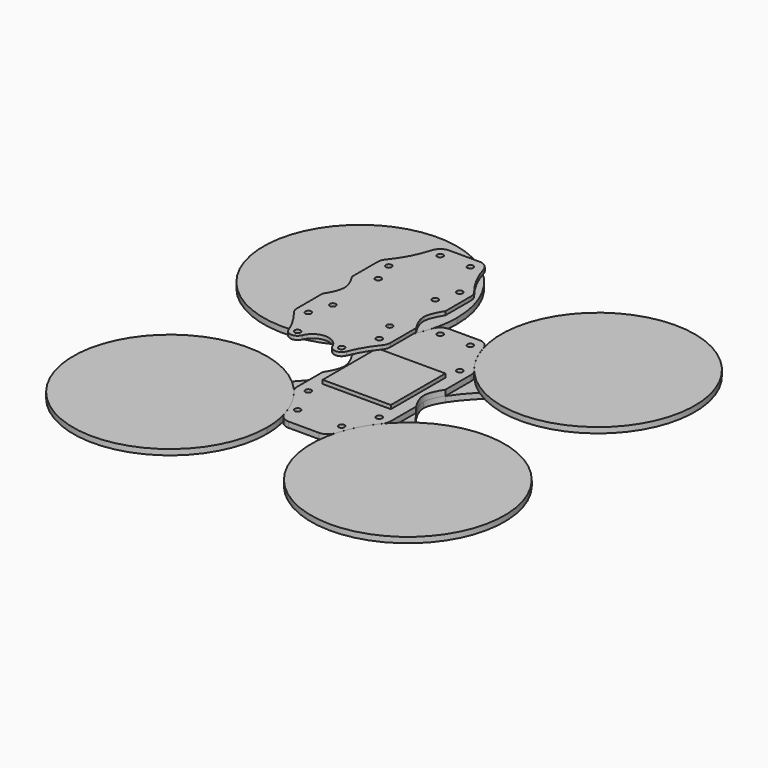
from build123d import *
from build123d import SkipClean  # not in build123d's __all__

# Parameters (mm, degrees)
F0_W      = 36.5
F0_H      = 20.4291760919
F0_H_2    = 36.5
F1_DEPTH  = 3
F2_DEPTH  = 5
F3_DEPTH  = 3
F5_DEPTH  = 3
F6_R      = 6
F8_DEPTH  = 3.001
F9_COUNT  = 2
F9_ANGLE  = 180
F12_DEPTH = 6.0010001
F14_R     = 1.6
F15_DEPTH = 6.0010001
F16_R     = 1.6
F17_DEPTH = 2
F20_DEPTH = 43.0010001


# Not quite as in the source:
# - the dataset's text gives a spline's control points without its knots; the knots are read off the source's solid
# - a pattern or mirror of a feature is missing from the dataset's text; its kind, count and spacing are read off the source's solid


with BuildPart() as f1:
    # F0 (on Top) → F1 (new body)
    with BuildSketch(Plane.XY):
        with BuildLine():
            ThreePointArc((18.25, 38.6791760919), (14.9470579592, 45.9682960976), (12.8062575721, 53.6791760919))
            Line((12.8062575721, 53.6791760919), (-12.8062575721, 53.6791760919))
            ThreePointArc((-12.8062575721, 53.6791760919), (-14.9470579592, 45.9682960976), (-18.25, 38.6791760919))
            Line((-18.25, 38.6791760919), (18.25, 38.6791760919))
        make_face()
        with Locations((0, 28.4645880459)):
            Rectangle(F0_W, F0_H)
        Rectangle(F0_W, F0_H_2)
        with Locations((0, -28.4645880459)):
            Rectangle(F0_W, F0_H)
        with BuildLine():
            ThreePointArc((12.8062575721, -53.6791760919), (14.9470579592, -45.9682960976), (18.25, -38.6791760919))
            Line((18.25, -38.6791760919), (-18.25, -38.6791760919))
            ThreePointArc((-18.25, -38.6791760919), (-14.9470579592, -45.9682960976), (-12.8062575721, -53.6791760919))
            Line((-12.8062575721, -53.6791760919), (12.8062575721, -53.6791760919))
        make_face()
        with BuildLine():
            Line((-18.25, 18.25), (-18.25, 38.6791760919))
            ThreePointArc((-18.25, 38.6791760919), (-21.3551418827, 33.7186522658), (-25, 29.1400376234))
            Line((-25, 29.1400376234), (-25, -29.1400376234))
            ThreePointArc((-25, -29.1400376234), (-21.3551418827, -33.7186522658), (-18.25, -38.6791760919))
            Line((-18.25, -38.6791760919), (-18.25, -18.25))
            Line((-18.25, -18.25), (-18.25, 18.25))
        make_face()
        with BuildLine():
            Line((25, -29.1400376234), (25, 29.1400376234))
            ThreePointArc((25, 29.1400376234), (21.3551418827, 33.7186522658), (18.25, 38.6791760919))
            Line((18.25, 38.6791760919), (18.25, 18.25))
            Line((18.25, 18.25), (18.25, -18.25))
            Line((18.25, -18.25), (18.25, -38.6791760919))
            ThreePointArc((18.25, -38.6791760919), (21.3551418827, -33.7186522658), (25, -29.1400376234))
        make_face()
    extrude(amount=F1_DEPTH)

    # F6
    f6_edges = [f1.edges().sort_by_distance(p)[0] for p in [
        (25, -29.140038, 1.5),
        (12.806258, -53.679176, 1.5),
        (25, 29.140038, 1.5),
        (12.806258, 53.679176, 1.5),
        (-12.806258, 53.679176, 1.5),
        (-25, 29.140038, 1.5),
        (-25, -29.140038, 1.5),
        (-12.806258, -53.679176, 1.5),
    ]]
    fillet(f6_edges, radius=F6_R)

    # F11 (on face) → F12 (cut, through all)
    with BuildSketch(Plane.XY.offset(3)):
        with BuildLine():
            Line((-25, 9.7909347539), (-25, -9.7909347533))
            add(Edge.make_bspline(
                [(-21.2132034356, 0), (-21.2132034356, -2.8448051924), (-22.673791932, -6.2126162774), (-24.9999999996, -9.7909347533)],
                knots=[0, 0, 0, 0, 0.1869288415, 0.1869288415, 0.1869288415, 0.1869288415], degree=3))
            add(Edge.make_bspline(
                [(-21.2132034356, 0), (-21.2132034356, 2.8448051925), (-22.6737919322, 6.2126162777), (-25, 9.7909347539)],
                knots=[0, 0, 0, 0, 0.1869288415, 0.1869288415, 0.1869288415, 0.1869288415], degree=3))
        make_face()
        with BuildLine():
            add(Edge.make_bspline(
                [(21.2132034356, 0), (21.2132034356, 2.8448051924), (22.673791932, 6.2126162774), (24.9999999996, 9.7909347533)],
                knots=[0, 0, 0, 0, 0.1869288415, 0.1869288415, 0.1869288415, 0.1869288415], degree=3))
            add(Edge.make_bspline(
                [(21.2132034356, 0), (21.2132034356, -2.8448051925), (22.6737919322, -6.2126162777), (25, -9.7909347539)],
                knots=[0, 0, 0, 0, 0.1869288415, 0.1869288415, 0.1869288415, 0.1869288415], degree=3))
            Line((25, -9.7909347539), (25, 9.7909347533))
        make_face()
    extrude(amount=-F12_DEPTH, mode=Mode.SUBTRACT)

    # F14 (on face) → F15 (cut, through all)
    with BuildSketch(Plane.XY.offset(3)):
        with Locations((19, 26.9225135853)):
            Circle(F14_R)
        with Locations((19, -26.9225135853)):
            Circle(F14_R)
        with Locations((8.0868917444, 47.6791760919)):
            Circle(F14_R)
        with Locations((15.25, 15.25)):
            Circle(F14_R)
        with Locations((15.25, -15.25)):
            Circle(F14_R)
        with Locations((11.7638554054, -43.0836852872)):
            Circle(F14_R)
    f15 = extrude(amount=-F15_DEPTH, mode=Mode.SUBTRACT)

    # F15_copies: F15 across plane
    add(f15.mirror(Plane(origin=(0, 0, 0), x_dir=(0, 0, -1), z_dir=(-1, 0, 0))), clean=False, mode=Mode.SUBTRACT)


with BuildPart() as f2:
    # F0 (on Top) → F2 (new body)
    with BuildSketch(Plane.XY):
        Rectangle(F0_W, F0_H_2)
    extrude(amount=F2_DEPTH)


with BuildPart() as f3:
    # F0 (on Top) → F3 (new body)
    with BuildSketch(Plane.XY):
        with BuildLine():
            Line((-25, 53.6791760919), (-12.8062575721, 53.6791760919))
            ThreePointArc((-12.8062575721, 53.6791760919), (-12.0818384792, 58.6359951966), (-11.8396103068, 63.6396103068))
            ThreePointArc((-11.8396103068, 63.6396103068), (-112.0378117914, 82.1018445447), (-25, 29.1400376234))
            Line((-25, 29.1400376234), (-25, 53.6791760919))
        make_face()
        with BuildLine():
            ThreePointArc((-18.25, 38.6791760919), (-14.9470579592, 45.9682960976), (-12.8062575721, 53.6791760919))
            Line((-12.8062575721, 53.6791760919), (-25, 53.6791760919))
            Line((-25, 53.6791760919), (-25, 29.1400376234))
            ThreePointArc((-25, 29.1400376234), (-21.3551418827, 33.7186522658), (-18.25, 38.6791760919))
        make_face()
    extrude(amount=F3_DEPTH)


with BuildPart() as f3b:
    # F0 (on Top) → F3, piece 2 (new body)
    with BuildSketch(Plane.XY):
        with BuildLine():
            ThreePointArc((25, 29.1400376234), (82.1018445447, 15.2414088222), (115.4396103068, 63.6396103068))
            ThreePointArc((115.4396103068, 63.6396103068), (58.6359951966, 115.1973821344), (12.8062575721, 53.6791760919))
            Line((12.8062575721, 53.6791760919), (25, 53.6791760919))
            Line((25, 53.6791760919), (25, 29.1400376234))
        make_face()
        with BuildLine():
            Line((25, 53.6791760919), (12.8062575721, 53.6791760919))
            ThreePointArc((12.8062575721, 53.6791760919), (14.9470579592, 45.9682960976), (18.25, 38.6791760919))
            ThreePointArc((18.25, 38.6791760919), (21.3551418827, 33.7186522658), (25, 29.1400376234))
            Line((25, 29.1400376234), (25, 53.6791760919))
        make_face()
    extrude(amount=F3_DEPTH)


with BuildPart() as f3c:
    # F0 (on Top) → F3, piece 3 (new body)
    with BuildSketch(Plane.XY):
        with BuildLine():
            Line((-25, -53.6791760919), (-25, -29.1400376234))
            ThreePointArc((-25, -29.1400376234), (-112.0378117914, -82.1018445447), (-11.8396103068, -63.6396103068))
            ThreePointArc((-11.8396103068, -63.6396103068), (-12.0818384792, -58.6359951966), (-12.8062575721, -53.6791760919))
            Line((-12.8062575721, -53.6791760919), (-25, -53.6791760919))
        make_face()
        with BuildLine():
            ThreePointArc((-12.8062575721, -53.6791760919), (-14.9470579592, -45.9682960976), (-18.25, -38.6791760919))
            ThreePointArc((-18.25, -38.6791760919), (-21.3551418827, -33.7186522658), (-25, -29.1400376234))
            Line((-25, -29.1400376234), (-25, -53.6791760919))
            Line((-25, -53.6791760919), (-12.8062575721, -53.6791760919))
        make_face()
    extrude(amount=F3_DEPTH)


with BuildPart() as f3d:
    # F0 (on Top) → F3, piece 4 (new body)
    with BuildSketch(Plane.XY):
        with BuildLine():
            ThreePointArc((115.4396103068, -63.6396103068), (82.1018445447, -15.2414088222), (25, -29.1400376234))
            Line((25, -29.1400376234), (25, -53.6791760919))
            Line((25, -53.6791760919), (12.8062575721, -53.6791760919))
            ThreePointArc((12.8062575721, -53.6791760919), (58.6359951966, -115.1973821344), (115.4396103068, -63.6396103068))
        make_face()
        with BuildLine():
            Line((25, -53.6791760919), (25, -29.1400376234))
            ThreePointArc((25, -29.1400376234), (21.3551418827, -33.7186522658), (18.25, -38.6791760919))
            ThreePointArc((18.25, -38.6791760919), (14.9470579592, -45.9682960976), (12.8062575721, -53.6791760919))
            Line((12.8062575721, -53.6791760919), (25, -53.6791760919))
        make_face()
    extrude(amount=F3_DEPTH)


with BuildPart() as f5:
    # F4 (on face) → F5 (new body)
    with BuildSketch(Plane.XY):
        with BuildLine():
            ThreePointArc((53.033008589, -74.2462120246), (74.2462120246, -74.2462120246), (74.2462120246, -53.033008589))
            Line((74.2462120246, -53.033008589), (21.2132034356, 0))
            Line((21.2132034356, 0), (0, 0))
            Line((0, 0), (0, -21.2132034356))
            Line((0, -21.2132034356), (53.033008589, -74.2462120246))
        make_face()
    extrude(amount=-F5_DEPTH)

    # F7 (on face) → F8 (cut, through all)
    with BuildSketch(Plane.XY):
        with BuildLine():
            add(Edge.make_bspline(
                [(25, -9.7909347539), (28.6766596733, -15.4466021988), (44.7457233208, -32.458147319), (59.4005470216, -44.1078131673), (70.4054520123, -50.2521764221)],
                knots=[0.1869288415, 0.1869288415, 0.1869288415, 0.1869288415, 0.4823769326, 1, 1, 1, 1], degree=3))
            ThreePointArc((70.4054520123, -50.2521764221), (72.4364111178, -51.4898656391), (74.2462120246, -53.033008589))
            Line((74.2462120246, -53.033008589), (25, -3.7867965644))
            Line((25, -3.7867965644), (25, -9.7909347539))
        make_face()
        with BuildLine():
            add(Edge.make_bspline(
                [(21.2132034356, 0), (21.2132034356, -2.8448051925), (22.6737919322, -6.2126162777), (25, -9.7909347539)],
                knots=[0, 0, 0, 0, 0.1869288415, 0.1869288415, 0.1869288415, 0.1869288415], degree=3))
            Line((25, -9.7909347539), (25, -3.7867965644))
            Line((25, -3.7867965644), (21.2132034356, 0))
        make_face()
    with SkipClean():  # cleaning this boolean's faces spoils the solid; the shape is the same uncleaned
        extrude(amount=-F8_DEPTH, mode=Mode.SUBTRACT)


with BuildPart() as f9_1:
    # F9: instance of F5
    add(f5.part.rotate(Axis((0, 0, -1.5), (0, 0, 1)), 1 * F9_ANGLE / (F9_COUNT - 1)), clean=False)


with BuildPart() as f10_1:
    # F10: instance of F9_1
    add(f9_1.part.mirror(Plane.YZ), clean=False)


with BuildPart() as f10_2:
    # F10: instance of F5
    add(f5.part.mirror(Plane.YZ), clean=False)


with BuildPart() as f17:
    # F16 (on offset) → F17 (new body)
    with BuildSketch(Plane.XY.offset(38)):
        with BuildLine():
            Line((25, -26.9225135853), (25, -9.7909347533))
            add(Edge.make_bspline(
                [(24.9999999996, -9.7909347533), (22.673791932, -6.2126162773), (21.2132034356, -2.8448051923), (21.2132034356, 0)],
                knots=[0.8130711585, 0.8130711585, 0.8130711585, 0.8130711585, 1, 1, 1, 1], degree=3))
            add(Edge.make_bspline(
                [(21.2132034356, 0), (21.2132034356, 2.8448051924), (22.673791932, 6.2126162774), (24.9999999996, 9.7909347533)],
                knots=[0, 0, 0, 0, 0.1869288415, 0.1869288415, 0.1869288415, 0.1869288415], degree=3))
            Line((25, 9.7909347533), (25, 26.9225135853))
            ThreePointArc((25, 26.9225135853), (24.6481509139, 28.9469619679), (23.633869582, 30.7339769128))
            ThreePointArc((23.633869582, 30.7339769128), (17.7904258459, 39.5337544981), (13.8536099343, 49.3359685709))
            ThreePointArc((13.8536099343, 49.3359685709), (11.6965485928, 52.4719182545), (8.0868917444, 53.6791760919))
            Line((8.0868917444, 53.6791760919), (-8.0868917444, 53.6791760919))
            ThreePointArc((-8.0868917444, 53.6791760919), (-11.6965485928, 52.4719182545), (-13.8536099343, 49.3359685709))
            ThreePointArc((-13.8536099343, 49.3359685709), (-17.7904258459, 39.5337544981), (-23.633869582, 30.7339769128))
            ThreePointArc((-23.633869582, 30.7339769128), (-24.6481509139, 28.9469619679), (-25, 26.9225135853))
            Line((-25, 26.9225135853), (-25, 9.790934753))
            add(Edge.make_bspline(
                [(-24.9999999996, 9.7909347533), (-22.673791932, 6.2126162773), (-21.2132034356, 2.8448051923), (-21.2132034356, 0)],
                knots=[0.8130711585, 0.8130711585, 0.8130711585, 0.8130711585, 1, 1, 1, 1], degree=3))
            add(Edge.make_bspline(
                [(-21.2132034356, 0), (-21.2132034356, -2.8448051924), (-22.673791932, -6.2126162774), (-24.9999999996, -9.7909347533)],
                knots=[0, 0, 0, 0, 0.1869288415, 0.1869288415, 0.1869288415, 0.1869288415], degree=3))
            Line((-25, -9.7909347533), (-25, -26.9225135853))
            ThreePointArc((-25, -26.9225135853), (-24.6481509139, -28.9469619679), (-23.633869582, -30.7339769128))
            ThreePointArc((-23.633869582, -30.7339769128), (-17.7904258459, -39.5337544981), (-13.8536099343, -49.3359685709))
            ThreePointArc((-13.8536099343, -49.3359685709), (-11.6965485928, -52.4719182545), (-8.0868917444, -53.6791760919))
            Line((-8.0868917444, -53.6791760919), (8.0868917444, -53.6791760919))
            ThreePointArc((8.0868917444, -53.6791760919), (11.6965485928, -52.4719182545), (13.8536099343, -49.3359685709))
            ThreePointArc((13.8536099343, -49.3359685709), (17.7904258459, -39.5337544981), (23.633869582, -30.7339769128))
            ThreePointArc((23.633869582, -30.7339769128), (24.6481509139, -28.9469619679), (25, -26.9225135853))
        make_face()
        with Locations((-19, -26.9225135853)):
            Circle(F16_R, mode=Mode.SUBTRACT)
        with Locations((-11.7638554054, -43.0836852872)):
            Circle(F16_R, mode=Mode.SUBTRACT)
        with Locations((-15.25, -15.25)):
            Circle(F16_R, mode=Mode.SUBTRACT)
        with Locations((11.7638554054, -43.0836852872)):
            Circle(F16_R, mode=Mode.SUBTRACT)
        with Locations((19, -26.9225135853)):
            Circle(F16_R, mode=Mode.SUBTRACT)
        with Locations((15.25, -15.25)):
            Circle(F16_R, mode=Mode.SUBTRACT)
        with Locations((-15.25, 15.25)):
            Circle(F16_R, mode=Mode.SUBTRACT)
        with Locations((-19, 26.9225135853)):
            Circle(F16_R, mode=Mode.SUBTRACT)
        with Locations((-8.0868917444, 47.6791760919)):
            Circle(F16_R, mode=Mode.SUBTRACT)
        with Locations((15.25, 15.25)):
            Circle(F16_R, mode=Mode.SUBTRACT)
        with Locations((8.0868917444, 47.6791760919)):
            Circle(F16_R, mode=Mode.SUBTRACT)
        with Locations((19, 26.9225135853)):
            Circle(F16_R, mode=Mode.SUBTRACT)
    extrude(amount=F17_DEPTH)

    # F19 (on face) → F20 (cut, through all)
    with BuildSketch(Plane.XY.offset(40)):
        with BuildLine():
            ThreePointArc((-7.9985502447, -44.433676786), (-11.6978293746, -47.0831403205), (-15.4825475216, -44.5572282776))
            ThreePointArc((-15.4825475216, -44.5572282776), (-14.6098234943, -46.9267408606), (-13.8536099343, -49.3359685709))
            ThreePointArc((-13.8536099343, -49.3359685709), (-11.6965485928, -52.4719182545), (-8.0868917444, -53.6791760919))
            Line((-8.0868917444, -53.6791760919), (8.0868917444, -53.6791760919))
            ThreePointArc((8.0868917444, -53.6791760919), (11.6965485928, -52.4719182545), (13.8536099343, -49.3359685709))
            ThreePointArc((13.8536099343, -49.3359685709), (14.609823496, -46.9267408558), (15.4825475253, -44.5572282683))
            ThreePointArc((15.4825475253, -44.5572282683), (11.6978293796, -47.0831403205), (7.9985502447, -44.433676786))
            ThreePointArc((7.9985502447, -44.433676786), (0, -39.1637810563), (-7.9985502447, -44.433676786))
        make_face()
    extrude(amount=-F20_DEPTH, mode=Mode.SUBTRACT)


solid = Compound([f1.part, f2.part, f3.part, f3b.part, f3c.part, f3d.part, f5.part, f9_1.part, f10_1.part, f10_2.part, f17.part])
